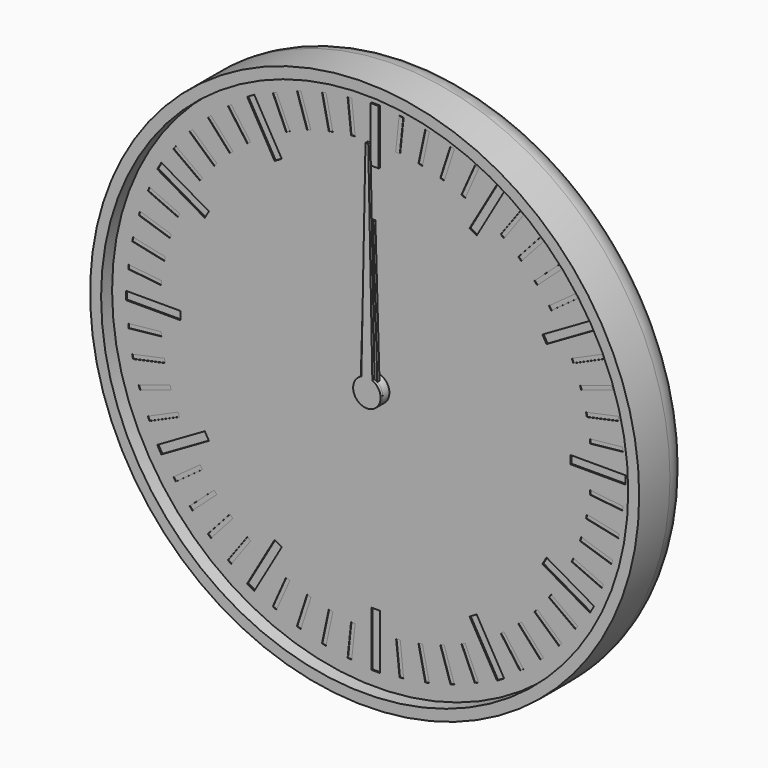
from build123d import *

# Parameters (mm, degrees)
F0_R      = 100
F1_DEPTH  = 24
F2_R      = 10
F3_T      = -4
F4_R      = 5
F4_R_2    = 3
F5_DEPTH  = 2
F6_DEPTH  = 19
F7_DEPTH  = 8
F9_DEPTH  = 4
F11_DEPTH = 4
F12_R     = 5
F12_R_2   = 3
F13_DEPTH = 2
F14_R     = 3
F15_DEPTH = 4
F17_DEPTH = 4
F18_R     = 3
F19_DEPTH = 2
F20_R     = 98
F20_R_2   = 5
F21_DEPTH = 1
F23_R     = 5
F23_R_2   = 3
F24_DEPTH = 2
F25_W     = 3
F25_H     = 20
F25_W_2   = 20
F25_H_2   = 3
F26_DEPTH = 0.5
F27_W     = 1.5
F27_H     = 12
F27_W_2   = 12
F27_H_2   = 1.5
F28_DEPTH = 0.2
F29_DEPTH = 1
F30_DEPTH = 0.4
F31_R     = 5
F31_R_2   = 3
F32_DEPTH = 5
F33_R     = 3
F34_DEPTH = 1
F36_DEPTH = 1


with BuildPart() as f1:
    # F0 (on Front) → F1 (new body)
    with BuildSketch(Plane.XZ):
        Circle(F0_R)
    extrude(amount=F1_DEPTH)

    # F2
    f2_edges = [f1.edges().sort_by_distance(p)[0] for p in [
        (-100, 0, 0),
    ]]
    fillet(f2_edges, radius=F2_R)

    # F3
    f3_openings = [f1.faces().sort_by_distance(p)[0] for p in [
        (0, -24, 0),
    ]]
    offset(amount=F3_T, openings=f3_openings)

    # F4 (on face) → F5 (join)
    with BuildSketch(Plane.XZ.offset(4)):
        Circle(F4_R)
        Circle(F4_R_2, mode=Mode.SUBTRACT)
        with Locations((40, 0)):
            Circle(F4_R)
        with Locations((40, 0)):
            Circle(F4_R_2, mode=Mode.SUBTRACT)
    extrude(amount=F5_DEPTH)


with BuildPart() as f6:
    # F6 (new): a face of the model
    f6_faces = [f1.part.faces().sort_by_distance(p)[0] for p in [
        (0, -4, 0),
    ]]
    extrude(f6_faces, amount=F6_DEPTH)

    # F8 (on face) → F9 (join)
    with BuildSketch(Plane.XZ.offset(6)):
        with BuildLine():
            ThreePointArc((9.2729637667, -1.3794085621), (9.3494561423, -0.6915886375), (9.375, 0))
            ThreePointArc((9.375, 0), (9.3494561423, 0.6915886375), (9.2729637667, 1.3794085621))
            ThreePointArc((9.2729637667, 1.3794085621), (8.9161548403, 2.8970343223), (8.3127812852, 4.3345463782))
            ThreePointArc((8.3127812852, 4.3345463782), (7.5845343223, 5.5104867402), (6.6911892658, 6.566476316))
            ThreePointArc((6.6911892658, 6.566476316), (5.5104867402, 7.5845343223), (4.1773988938, 8.3928519278))
            ThreePointArc((4.1773988938, 8.3928519278), (2.8970343223, 8.9161548403), (1.5536078905, 9.2453733036))
            ThreePointArc((1.5536078905, 9.2453733036), (0, 9.375), (-1.5536078905, 9.2453733036))
            ThreePointArc((-1.5536078905, 9.2453733036), (-2.8970343223, 8.9161548403), (-4.1773988938, 8.3928519278))
            ThreePointArc((-4.1773988938, 8.3928519278), (-5.5104867402, 7.5845343223), (-6.6911892658, 6.566476316))
            ThreePointArc((-6.6911892658, 6.566476316), (-7.5845343223, 5.5104867402), (-8.3127812852, 4.3345463782))
            ThreePointArc((-8.3127812852, 4.3345463782), (-8.9161548403, 2.8970343223), (-9.2729637667, 1.3794085621))
            ThreePointArc((-9.2729637667, 1.3794085621), (-9.375, 0), (-9.2729637667, -1.3794085621))
            ThreePointArc((-9.2729637667, -1.3794085621), (-8.9161548403, -2.8970343223), (-8.3127812852, -4.3345463782))
            ThreePointArc((-8.3127812852, -4.3345463782), (-7.5845343223, -5.5104867402), (-6.6911892658, -6.566476316))
            ThreePointArc((-6.6911892658, -6.566476316), (-5.5104867402, -7.5845343223), (-4.1773988938, -8.3928519278))
            ThreePointArc((-4.1773988938, -8.3928519278), (-2.8970343223, -8.9161548403), (-1.5536078905, -9.2453733036))
            ThreePointArc((-1.5536078905, -9.2453733036), (0, -9.375), (1.5536078905, -9.2453733036))
            ThreePointArc((1.5536078905, -9.2453733036), (2.8970343223, -8.9161548403), (4.1773988938, -8.3928519278))
            ThreePointArc((4.1773988938, -8.3928519278), (5.5104867402, -7.5845343223), (6.6911892658, -6.566476316))
            ThreePointArc((6.6911892658, -6.566476316), (7.5845343223, -5.5104867402), (8.3127812852, -4.3345463782))
            ThreePointArc((8.3127812852, -4.3345463782), (8.9161548403, -2.8970343223), (9.2729637667, -1.3794085621))
        make_face()
        with BuildLine():
            ThreePointArc((8.3127812852, 4.3345463782), (8.9161548403, 2.8970343223), (9.2729637667, 1.3794085621))
            Line((9.2729637667, 1.3794085621), (11.1823199426, 2.3946312492))
            Line((11.1823199426, 2.3946312492), (10.8182678729, 3.515068311))
            Line((10.8182678729, 3.515068311), (10.4542158031, 4.6355053728))
            Line((10.4542158031, 4.6355053728), (8.3127812852, 4.3345463782))
        make_face()
        with BuildLine():
            Line((11.1823199426, -2.3946312492), (9.2729637667, -1.3794085621))
            ThreePointArc((9.2729637667, -1.3794085621), (8.9161548403, -2.8970343223), (8.3127812852, -4.3345463782))
            Line((8.3127812852, -4.3345463782), (10.4542158031, -4.6355053728))
            Line((10.4542158031, -4.6355053728), (10.8182678729, -3.515068311))
            Line((10.8182678729, -3.515068311), (11.1823199426, -2.3946312492))
        make_face()
        with BuildLine():
            ThreePointArc((4.1773988938, 8.3928519278), (5.5104867402, 7.5845343223), (6.6911892658, 6.566476316))
            Line((6.6911892658, 6.566476316), (7.6391579371, 8.5101001246))
            Line((7.6391579371, 8.5101001246), (6.6860572448, 9.202568311))
            Line((6.6860572448, 9.202568311), (5.7329565525, 9.8950364974))
            Line((5.7329565525, 9.8950364974), (4.1773988938, 8.3928519278))
        make_face()
        with BuildLine():
            Line((7.6391579371, -8.5101001246), (6.6911892658, -6.566476316))
            ThreePointArc((6.6911892658, -6.566476316), (5.5104867402, -7.5845343223), (4.1773988938, -8.3928519278))
            Line((4.1773988938, -8.3928519278), (5.7329565525, -9.8950364974))
            Line((5.7329565525, -9.8950364974), (6.6860572448, -9.202568311))
            Line((6.6860572448, -9.202568311), (7.6391579371, -8.5101001246))
        make_face()
        with BuildLine():
            ThreePointArc((-1.5536078905, 9.2453733036), (0, 9.375), (1.5536078905, 9.2453733036))
            Line((1.5536078905, 9.2453733036), (1.1780972451, 11.375))
            Line((1.1780972451, 11.375), (0, 11.375))
            Line((0, 11.375), (-1.1780972451, 11.375))
            Line((-1.1780972451, 11.375), (-1.5536078905, 9.2453733036))
        make_face()
        with BuildLine():
            Line((1.1780972451, -11.375), (1.5536078905, -9.2453733036))
            ThreePointArc((1.5536078905, -9.2453733036), (0, -9.375), (-1.5536078905, -9.2453733036))
            Line((-1.5536078905, -9.2453733036), (-1.1780972451, -11.375))
            Line((-1.1780972451, -11.375), (0, -11.375))
            Line((0, -11.375), (1.1780972451, -11.375))
        make_face()
        with BuildLine():
            ThreePointArc((-6.6911892658, 6.566476316), (-5.5104867402, 7.5845343223), (-4.1773988938, 8.3928519278))
            Line((-4.1773988938, 8.3928519278), (-5.7329565525, 9.8950364974))
            Line((-5.7329565525, 9.8950364974), (-6.6860572448, 9.202568311))
            Line((-6.6860572448, 9.202568311), (-7.6391579371, 8.5101001246))
            Line((-7.6391579371, 8.5101001246), (-6.6911892658, 6.566476316))
        make_face()
        with BuildLine():
            Line((-5.7329565525, -9.8950364974), (-4.1773988938, -8.3928519278))
            ThreePointArc((-4.1773988938, -8.3928519278), (-5.5104867402, -7.5845343223), (-6.6911892658, -6.566476316))
            Line((-6.6911892658, -6.566476316), (-7.6391579371, -8.5101001246))
            Line((-7.6391579371, -8.5101001246), (-6.6860572448, -9.202568311))
            Line((-6.6860572448, -9.202568311), (-5.7329565525, -9.8950364974))
        make_face()
        with BuildLine():
            ThreePointArc((-9.2729637667, 1.3794085621), (-8.9161548403, 2.8970343223), (-8.3127812852, 4.3345463782))
            Line((-8.3127812852, 4.3345463782), (-10.4542158031, 4.6355053728))
            Line((-10.4542158031, 4.6355053728), (-10.8182678729, 3.515068311))
            Line((-10.8182678729, 3.515068311), (-11.1823199426, 2.3946312492))
            Line((-11.1823199426, 2.3946312492), (-9.2729637667, 1.3794085621))
        make_face()
        with BuildLine():
            Line((-10.4542158031, -4.6355053728), (-8.3127812852, -4.3345463782))
            ThreePointArc((-8.3127812852, -4.3345463782), (-8.9161548403, -2.8970343223), (-9.2729637667, -1.3794085621))
            Line((-9.2729637667, -1.3794085621), (-11.1823199426, -2.3946312492))
            Line((-11.1823199426, -2.3946312492), (-10.8182678729, -3.515068311))
            Line((-10.8182678729, -3.515068311), (-10.4542158031, -4.6355053728))
        make_face()
    extrude(amount=F9_DEPTH)

    # F35 (on face) → F36 (join)
    with BuildSketch(Plane.XZ.offset(23)):
        with BuildLine():
            ThreePointArc((-2, 4.582575695), (-2.7386127875, -4.1833001327), (5, 0))
            ThreePointArc((5, 0), (4.1833001327, 2.7386127875), (2, 4.582575695))
            ThreePointArc((2, 4.582575695), (0, 5), (-2, 4.582575695))
        make_face()
        with BuildLine():
            ThreePointArc((-2, 4.582575695), (0, 5), (2, 4.582575695))
            Line((2, 4.582575695), (0.5, 80))
            Line((0.5, 80), (0, 80))
            Line((0, 80), (-0.5, 80))
            Line((-0.5, 80), (-2, 4.582575695))
        make_face()
    extrude(amount=-F36_DEPTH)


with BuildPart() as f7:
    # F7 (new): a face of the model
    f7_faces = [f1.part.faces().sort_by_distance(p)[0] for p in [
        (40, -4, 0),
    ]]
    extrude(f7_faces, amount=F7_DEPTH)

    # F10 (on face) → F11 (join)
    with BuildSketch(Plane.XZ.offset(6)):
        with BuildLine():
            ThreePointArc((68.0829066802, -1.5381733945), (68.1144747006, -0.7693746225), (68.125, 0))
            ThreePointArc((68.125, 0), (68.1144747006, 0.7693746225), (68.0829066802, 1.5381733945))
            ThreePointArc((68.0829066802, 1.5381733945), (67.9709283072, 2.9398630294), (67.7890320221, 4.3342039956))
            ThreePointArc((67.7890320221, 4.3342039956), (67.5104012706, 5.8475163042), (67.1494235596, 7.3433252263))
            ThreePointArc((67.1494235596, 7.3433252263), (66.7484645208, 8.6911029668), (66.280643318, 10.0171558733))
            ThreePointArc((66.280643318, 10.0171558733), (65.6934659962, 11.4394680865), (65.0293803521, 12.8275385085))
            ThreePointArc((65.0293803521, 12.8275385085), (64.3569644814, 14.0625), (63.6236643925, 15.2623099717))
            ThreePointArc((63.6236643925, 15.2623099717), (62.7536029668, 16.5314602207), (61.815433119, 17.7511268046))
            ThreePointArc((61.815433119, 17.7511268046), (60.9009482166, 18.8192983038), (59.934217974, 19.8404278876))
            ThreePointArc((59.934217974, 19.8404278876), (58.8192983038, 20.9009482166), (57.6480467764, 21.8989056799))
            ThreePointArc((57.6480467764, 21.8989056799), (56.5314602207, 22.7536029668), (55.3735505752, 23.5514238999))
            ThreePointArc((55.3735505752, 23.5514238999), (54.0625, 24.3569644814), (52.709356105, 25.0895972944))
            ThreePointArc((52.709356105, 25.0895972944), (51.4394680865, 25.6934659962), (50.1409852457, 26.2331096755))
            ThreePointArc((50.1409852457, 26.2331096755), (48.6911029668, 26.7484645208), (47.2152055856, 27.1837531139))
            ThreePointArc((47.2152055856, 27.1837531139), (45.8475163042, 27.5104012706), (44.4652101991, 27.7682826779))
            ThreePointArc((44.4652101991, 27.7682826779), (42.9398630294, 27.9709283072), (41.4057159597, 28.0898484802))
            ThreePointArc((41.4057159597, 28.0898484802), (40, 28.125), (38.5942840403, 28.0898484802))
            ThreePointArc((38.5942840403, 28.0898484802), (37.0601369706, 27.9709283072), (35.5347898009, 27.7682826779))
            ThreePointArc((35.5347898009, 27.7682826779), (34.1524836958, 27.5104012706), (32.7847944144, 27.1837531139))
            ThreePointArc((32.7847944144, 27.1837531139), (31.3088970332, 26.7484645208), (29.8590147543, 26.2331096755))
            ThreePointArc((29.8590147543, 26.2331096755), (28.5605319135, 25.6934659962), (27.290643895, 25.0895972944))
            ThreePointArc((27.290643895, 25.0895972944), (25.9375, 24.3569644814), (24.6264494248, 23.5514238999))
            ThreePointArc((24.6264494248, 23.5514238999), (23.4685397793, 22.7536029668), (22.3519532236, 21.8989056799))
            ThreePointArc((22.3519532236, 21.8989056799), (21.1807016962, 20.9009482166), (20.065782026, 19.8404278876))
            ThreePointArc((20.065782026, 19.8404278876), (19.0990517834, 18.8192983038), (18.184566881, 17.7511268046))
            ThreePointArc((18.184566881, 17.7511268046), (17.2463970332, 16.5314602207), (16.3763356075, 15.2623099717))
            ThreePointArc((16.3763356075, 15.2623099717), (15.6430355186, 14.0625), (14.9706196479, 12.8275385085))
            ThreePointArc((14.9706196479, 12.8275385085), (14.3065340038, 11.4394680865), (13.719356682, 10.0171558733))
            ThreePointArc((13.719356682, 10.0171558733), (13.2515354792, 8.6911029668), (12.8505764404, 7.3433252263))
            ThreePointArc((12.8505764404, 7.3433252263), (12.4895987294, 5.8475163042), (12.2109679779, 4.3342039956))
            ThreePointArc((12.2109679779, 4.3342039956), (12.0290716928, 2.9398630294), (11.9170933198, 1.5381733945))
            ThreePointArc((11.9170933198, 1.5381733945), (11.875, 0), (11.9170933198, -1.5381733945))
            ThreePointArc((11.9170933198, -1.5381733945), (12.0290716928, -2.9398630294), (12.2109679779, -4.3342039956))
            ThreePointArc((12.2109679779, -4.3342039956), (12.4895987294, -5.8475163042), (12.8505764404, -7.3433252263))
            ThreePointArc((12.8505764404, -7.3433252263), (13.2515354792, -8.6911029668), (13.719356682, -10.0171558733))
            ThreePointArc((13.719356682, -10.0171558733), (14.3065340038, -11.4394680865), (14.9706196479, -12.8275385085))
            ThreePointArc((14.9706196479, -12.8275385085), (15.6430355186, -14.0625), (16.3763356075, -15.2623099717))
            ThreePointArc((16.3763356075, -15.2623099717), (17.2463970332, -16.5314602207), (18.184566881, -17.7511268046))
            ThreePointArc((18.184566881, -17.7511268046), (19.0990517834, -18.8192983038), (20.065782026, -19.8404278876))
            ThreePointArc((20.065782026, -19.8404278876), (21.1807016962, -20.9009482166), (22.3519532236, -21.8989056799))
            ThreePointArc((22.3519532236, -21.8989056799), (23.4685397793, -22.7536029668), (24.6264494248, -23.5514238999))
            ThreePointArc((24.6264494248, -23.5514238999), (25.9375, -24.3569644814), (27.290643895, -25.0895972944))
            ThreePointArc((27.290643895, -25.0895972944), (28.5605319135, -25.6934659962), (29.8590147543, -26.2331096755))
            ThreePointArc((29.8590147543, -26.2331096755), (31.3088970332, -26.7484645208), (32.7847944144, -27.1837531139))
            ThreePointArc((32.7847944144, -27.1837531139), (34.1524836958, -27.5104012706), (35.5347898009, -27.7682826779))
            ThreePointArc((35.5347898009, -27.7682826779), (37.0601369706, -27.9709283072), (38.5942840403, -28.0898484802))
            ThreePointArc((38.5942840403, -28.0898484802), (40, -28.125), (41.4057159597, -28.0898484802))
            ThreePointArc((41.4057159597, -28.0898484802), (42.9398630294, -27.9709283072), (44.4652101991, -27.7682826779))
            ThreePointArc((44.4652101991, -27.7682826779), (45.8475163042, -27.5104012706), (47.2152055856, -27.1837531139))
            ThreePointArc((47.2152055856, -27.1837531139), (48.6911029668, -26.7484645208), (50.1409852457, -26.2331096755))
            ThreePointArc((50.1409852457, -26.2331096755), (51.4394680865, -25.6934659962), (52.709356105, -25.0895972944))
            ThreePointArc((52.709356105, -25.0895972944), (54.0625, -24.3569644814), (55.3735505752, -23.5514238999))
            ThreePointArc((55.3735505752, -23.5514238999), (56.5314602207, -22.7536029668), (57.6480467764, -21.8989056799))
            ThreePointArc((57.6480467764, -21.8989056799), (58.8192983038, -20.9009482166), (59.934217974, -19.8404278876))
            ThreePointArc((59.934217974, -19.8404278876), (60.9009482166, -18.8192983038), (61.815433119, -17.7511268046))
            ThreePointArc((61.815433119, -17.7511268046), (62.7536029668, -16.5314602207), (63.6236643925, -15.2623099717))
            ThreePointArc((63.6236643925, -15.2623099717), (64.3569644814, -14.0625), (65.0293803521, -12.8275385085))
            ThreePointArc((65.0293803521, -12.8275385085), (65.6934659962, -11.4394680865), (66.280643318, -10.0171558733))
            ThreePointArc((66.280643318, -10.0171558733), (66.7484645208, -8.6911029668), (67.1494235596, -7.3433252263))
            ThreePointArc((67.1494235596, -7.3433252263), (67.5104012706, -5.8475163042), (67.7890320221, -4.3342039956))
            ThreePointArc((67.7890320221, -4.3342039956), (67.9709283072, -2.9398630294), (68.0829066802, -1.5381733945))
        make_face()
        with BuildLine():
            ThreePointArc((68.0829066802, 1.5381733945), (68.1144747006, 0.7693746225), (68.125, 0))
            ThreePointArc((68.125, 0), (68.1144747006, -0.7693746225), (68.0829066802, -1.5381733945))
            Line((68.0829066802, -1.5381733945), (70.125, -1.1780972451))
            Line((70.125, -1.1780972451), (70.125, 0))
            Line((70.125, 0), (70.125, 1.1780972451))
            Line((70.125, 1.1780972451), (68.0829066802, 1.5381733945))
        make_face()
        with BuildLine():
            ThreePointArc((67.1494235596, 7.3433252263), (67.5104012706, 5.8475163042), (67.7890320221, 4.3342039956))
            Line((67.7890320221, 4.3342039956), (69.7116366623, 5.1109866922))
            Line((69.7116366623, 5.1109866922), (69.4666964721, 6.2633396859))
            Line((69.4666964721, 6.2633396859), (69.2217562819, 7.4156926796))
            Line((69.2217562819, 7.4156926796), (67.1494235596, 7.3433252263))
        make_face()
        with BuildLine():
            Line((69.7116366623, -5.1109866922), (67.7890320221, -4.3342039956))
            ThreePointArc((67.7890320221, -4.3342039956), (67.5104012706, -5.8475163042), (67.1494235596, -7.3433252263))
            Line((67.1494235596, -7.3433252263), (69.2217562819, -7.4156926796))
            Line((69.2217562819, -7.4156926796), (69.4666964721, -6.2633396859))
            Line((69.4666964721, -6.2633396859), (69.7116366623, -5.1109866922))
        make_face()
        with BuildLine():
            ThreePointArc((65.0293803521, 12.8275385085), (65.6934659962, 11.4394680865), (66.280643318, 10.0171558733))
            Line((66.280643318, 10.0171558733), (67.9997322302, 11.1766959857))
            Line((67.9997322302, 11.1766959857), (67.5205569115, 12.2529413727))
            Line((67.5205569115, 12.2529413727), (67.0413815928, 13.3291867596))
            Line((67.0413815928, 13.3291867596), (65.0293803521, 12.8275385085))
        make_face()
        with BuildLine():
            Line((67.9997322302, -11.1766959857), (66.280643318, -10.0171558733))
            ThreePointArc((66.280643318, -10.0171558733), (65.6934659962, -11.4394680865), (65.0293803521, -12.8275385085))
            Line((65.0293803521, -12.8275385085), (67.0413815928, -13.3291867596))
            Line((67.0413815928, -13.3291867596), (67.5205569115, -12.2529413727))
            Line((67.5205569115, -12.2529413727), (67.9997322302, -11.1766959857))
        make_face()
        with BuildLine():
            ThreePointArc((61.815433119, 17.7511268046), (62.7536029668, 16.5314602207), (63.6236643925, 15.2623099717))
            Line((63.6236643925, 15.2623099717), (65.064105142, 16.753930033))
            Line((65.064105142, 16.753930033), (64.3716369555, 17.7070307253))
            Line((64.3716369555, 17.7070307253), (63.6791687691, 18.6601314176))
            Line((63.6791687691, 18.6601314176), (61.815433119, 17.7511268046))
        make_face()
        with BuildLine():
            Line((65.064105142, -16.753930033), (63.6236643925, -15.2623099717))
            ThreePointArc((63.6236643925, -15.2623099717), (62.7536029668, -16.5314602207), (61.815433119, -17.7511268046))
            Line((61.815433119, -17.7511268046), (63.6791687691, -18.6601314176))
            Line((63.6791687691, -18.6601314176), (64.3716369555, -17.7070307253))
            Line((64.3716369555, -17.7070307253), (65.064105142, -16.753930033))
        make_face()
        with BuildLine():
            ThreePointArc((57.6480467764, 21.8989056799), (58.8192983038, 20.9009482166), (59.934217974, 19.8404278876))
            Line((59.934217974, 19.8404278876), (61.0330563882, 21.5989369435))
            Line((61.0330563882, 21.5989369435), (60.1575595166, 22.3872378675))
            Line((60.1575595166, 22.3872378675), (59.282062645, 23.1755387915))
            Line((59.282062645, 23.1755387915), (57.6480467764, 21.8989056799))
        make_face()
        with BuildLine():
            Line((61.0330563882, -21.5989369435), (59.934217974, -19.8404278876))
            ThreePointArc((59.934217974, -19.8404278876), (58.8192983038, -20.9009482166), (57.6480467764, -21.8989056799))
            Line((57.6480467764, -21.8989056799), (59.282062645, -23.1755387915))
            Line((59.282062645, -23.1755387915), (60.1575595166, -22.3872378675))
            Line((60.1575595166, -22.3872378675), (61.0330563882, -21.5989369435))
        make_face()
        with BuildLine():
            ThreePointArc((52.709356105, 25.0895972944), (54.0625, 24.3569644814), (55.3735505752, 23.5514238999))
            Line((55.3735505752, 23.5514238999), (56.0827621424, 25.4999666665))
            Line((56.0827621424, 25.4999666665), (55.0625, 26.089015289))
            Line((55.0625, 26.089015289), (54.0422378576, 26.6780639116))
            Line((54.0422378576, 26.6780639116), (52.709356105, 25.0895972944))
        make_face()
        with BuildLine():
            Line((56.0827621424, -25.4999666665), (55.3735505752, -23.5514238999))
            ThreePointArc((55.3735505752, -23.5514238999), (54.0625, -24.3569644814), (52.709356105, -25.0895972944))
            Line((52.709356105, -25.0895972944), (54.0422378576, -26.6780639116))
            Line((54.0422378576, -26.6780639116), (55.0625, -26.089015289))
            Line((55.0625, -26.089015289), (56.0827621424, -25.4999666665))
        make_face()
        with BuildLine():
            ThreePointArc((47.2152055856, 27.1837531139), (48.6911029668, 26.7484645208), (50.1409852457, 26.2331096755))
            Line((50.1409852457, 26.2331096755), (50.4295740173, 28.2865254836))
            Line((50.4295740173, 28.2865254836), (49.3091369555, 28.6505775534))
            Line((49.3091369555, 28.6505775534), (48.1886998938, 29.0146296232))
            Line((48.1886998938, 29.0146296232), (47.2152055856, 27.1837531139))
        make_face()
        with BuildLine():
            Line((50.4295740173, -28.2865254836), (50.1409852457, -26.2331096755))
            ThreePointArc((50.1409852457, -26.2331096755), (48.6911029668, -26.7484645208), (47.2152055856, -27.1837531139))
            Line((47.2152055856, -27.1837531139), (48.1886998938, -29.0146296232))
            Line((48.1886998938, -29.0146296232), (49.3091369555, -28.6505775534))
            Line((49.3091369555, -28.6505775534), (50.4295740173, -28.2865254836))
        make_face()
        with BuildLine():
            ThreePointArc((41.4057159597, 28.0898484802), (42.9398630294, 27.9709283072), (44.4652101991, 27.7682826779))
            Line((44.4652101991, 27.7682826779), (44.3205634611, 29.8368274034))
            Line((44.3205634611, 29.8368274034), (43.1489199559, 29.959972098))
            Line((43.1489199559, 29.959972098), (41.9772764508, 30.0831167926))
            Line((41.9772764508, 30.0831167926), (41.4057159597, 28.0898484802))
        make_face()
        with BuildLine():
            Line((44.3205634611, -29.8368274034), (44.4652101991, -27.7682826779))
            ThreePointArc((44.4652101991, -27.7682826779), (42.9398630294, -27.9709283072), (41.4057159597, -28.0898484802))
            Line((41.4057159597, -28.0898484802), (41.9772764508, -30.0831167926))
            Line((41.9772764508, -30.0831167926), (43.1489199559, -29.959972098))
            Line((43.1489199559, -29.959972098), (44.3205634611, -29.8368274034))
        make_face()
        with BuildLine():
            ThreePointArc((35.5347898009, 27.7682826779), (37.0601369706, 27.9709283072), (38.5942840403, 28.0898484802))
            Line((38.5942840403, 28.0898484802), (38.0227235492, 30.0831167926))
            Line((38.0227235492, 30.0831167926), (36.8510800441, 29.959972098))
            Line((36.8510800441, 29.959972098), (35.6794365389, 29.8368274034))
            Line((35.6794365389, 29.8368274034), (35.5347898009, 27.7682826779))
        make_face()
        with BuildLine():
            Line((38.0227235492, -30.0831167926), (38.5942840403, -28.0898484802))
            ThreePointArc((38.5942840403, -28.0898484802), (37.0601369706, -27.9709283072), (35.5347898009, -27.7682826779))
            Line((35.5347898009, -27.7682826779), (35.6794365389, -29.8368274034))
            Line((35.6794365389, -29.8368274034), (36.8510800441, -29.959972098))
            Line((36.8510800441, -29.959972098), (38.0227235492, -30.0831167926))
        make_face()
        with BuildLine():
            ThreePointArc((29.8590147543, 26.2331096755), (31.3088970332, 26.7484645208), (32.7847944144, 27.1837531139))
            Line((32.7847944144, 27.1837531139), (31.8113001062, 29.0146296232))
            Line((31.8113001062, 29.0146296232), (30.6908630445, 28.6505775534))
            Line((30.6908630445, 28.6505775534), (29.5704259827, 28.2865254836))
            Line((29.5704259827, 28.2865254836), (29.8590147543, 26.2331096755))
        make_face()
        with BuildLine():
            Line((31.8113001062, -29.0146296232), (32.7847944144, -27.1837531139))
            ThreePointArc((32.7847944144, -27.1837531139), (31.3088970332, -26.7484645208), (29.8590147543, -26.2331096755))
            Line((29.8590147543, -26.2331096755), (29.5704259827, -28.2865254836))
            Line((29.5704259827, -28.2865254836), (30.6908630445, -28.6505775534))
            Line((30.6908630445, -28.6505775534), (31.8113001062, -29.0146296232))
        make_face()
        with BuildLine():
            ThreePointArc((24.6264494248, 23.5514238999), (25.9375, 24.3569644814), (27.290643895, 25.0895972944))
            Line((27.290643895, 25.0895972944), (25.9577621424, 26.6780639116))
            Line((25.9577621424, 26.6780639116), (24.9375, 26.089015289))
            Line((24.9375, 26.089015289), (23.9172378576, 25.4999666665))
            Line((23.9172378576, 25.4999666665), (24.6264494248, 23.5514238999))
        make_face()
        with BuildLine():
            Line((25.9577621424, -26.6780639116), (27.290643895, -25.0895972944))
            ThreePointArc((27.290643895, -25.0895972944), (25.9375, -24.3569644814), (24.6264494248, -23.5514238999))
            Line((24.6264494248, -23.5514238999), (23.9172378576, -25.4999666665))
            Line((23.9172378576, -25.4999666665), (24.9375, -26.089015289))
            Line((24.9375, -26.089015289), (25.9577621424, -26.6780639116))
        make_face()
        with BuildLine():
            ThreePointArc((20.065782026, 19.8404278876), (21.1807016962, 20.9009482166), (22.3519532236, 21.8989056799))
            Line((22.3519532236, 21.8989056799), (20.717937355, 23.1755387915))
            Line((20.717937355, 23.1755387915), (19.8424404834, 22.3872378675))
            Line((19.8424404834, 22.3872378675), (18.9669436118, 21.5989369435))
            Line((18.9669436118, 21.5989369435), (20.065782026, 19.8404278876))
        make_face()
        with BuildLine():
            Line((20.717937355, -23.1755387915), (22.3519532236, -21.8989056799))
            ThreePointArc((22.3519532236, -21.8989056799), (21.1807016962, -20.9009482166), (20.065782026, -19.8404278876))
            Line((20.065782026, -19.8404278876), (18.9669436118, -21.5989369435))
            Line((18.9669436118, -21.5989369435), (19.8424404834, -22.3872378675))
            Line((19.8424404834, -22.3872378675), (20.717937355, -23.1755387915))
        make_face()
        with BuildLine():
            ThreePointArc((16.3763356075, 15.2623099717), (17.2463970332, 16.5314602207), (18.184566881, 17.7511268046))
            Line((18.184566881, 17.7511268046), (16.3208312309, 18.6601314176))
            Line((16.3208312309, 18.6601314176), (15.6283630445, 17.7070307253))
            Line((15.6283630445, 17.7070307253), (14.935894858, 16.753930033))
            Line((14.935894858, 16.753930033), (16.3763356075, 15.2623099717))
        make_face()
        with BuildLine():
            Line((16.3208312309, -18.6601314176), (18.184566881, -17.7511268046))
            ThreePointArc((18.184566881, -17.7511268046), (17.2463970332, -16.5314602207), (16.3763356075, -15.2623099717))
            Line((16.3763356075, -15.2623099717), (14.935894858, -16.753930033))
            Line((14.935894858, -16.753930033), (15.6283630445, -17.7070307253))
            Line((15.6283630445, -17.7070307253), (16.3208312309, -18.6601314176))
        make_face()
        with BuildLine():
            ThreePointArc((13.719356682, 10.0171558733), (14.3065340038, 11.4394680865), (14.9706196479, 12.8275385085))
            Line((14.9706196479, 12.8275385085), (12.9586184072, 13.3291867596))
            Line((12.9586184072, 13.3291867596), (12.4794430885, 12.2529413727))
            Line((12.4794430885, 12.2529413727), (12.0002677698, 11.1766959857))
            Line((12.0002677698, 11.1766959857), (13.719356682, 10.0171558733))
        make_face()
        with BuildLine():
            Line((12.9586184072, -13.3291867596), (14.9706196479, -12.8275385085))
            ThreePointArc((14.9706196479, -12.8275385085), (14.3065340038, -11.4394680865), (13.719356682, -10.0171558733))
            Line((13.719356682, -10.0171558733), (12.0002677698, -11.1766959857))
            Line((12.0002677698, -11.1766959857), (12.4794430885, -12.2529413727))
            Line((12.4794430885, -12.2529413727), (12.9586184072, -13.3291867596))
        make_face()
        with BuildLine():
            ThreePointArc((12.2109679779, 4.3342039956), (12.4895987294, 5.8475163042), (12.8505764404, 7.3433252263))
            Line((12.8505764404, 7.3433252263), (10.7782437181, 7.4156926796))
            Line((10.7782437181, 7.4156926796), (10.5333035279, 6.2633396859))
            Line((10.5333035279, 6.2633396859), (10.2883633377, 5.1109866922))
            Line((10.2883633377, 5.1109866922), (12.2109679779, 4.3342039956))
        make_face()
        with BuildLine():
            Line((10.7782437181, -7.4156926796), (12.8505764404, -7.3433252263))
            ThreePointArc((12.8505764404, -7.3433252263), (12.4895987294, -5.8475163042), (12.2109679779, -4.3342039956))
            Line((12.2109679779, -4.3342039956), (10.2883633377, -5.1109866922))
            Line((10.2883633377, -5.1109866922), (10.5333035279, -6.2633396859))
            Line((10.5333035279, -6.2633396859), (10.7782437181, -7.4156926796))
        make_face()
        with BuildLine():
            ThreePointArc((11.9170933198, -1.5381733945), (11.875, 0), (11.9170933198, 1.5381733945))
            Line((11.9170933198, 1.5381733945), (9.875, 1.1780972451))
            Line((9.875, 1.1780972451), (9.875, 0))
            Line((9.875, 0), (9.875, -1.1780972451))
            Line((9.875, -1.1780972451), (11.9170933198, -1.5381733945))
        make_face()
    extrude(amount=F11_DEPTH)

    # F16 (on face) → F17 (join)
    with BuildSketch(Plane.XZ.offset(12)):
        with BuildLine():
            ThreePointArc((47.4288750323, -1.0304444454), (47.4821976298, -0.5164480894), (47.5, 0))
            ThreePointArc((47.5, 0), (47.4821976298, 0.5164480894), (47.4288750323, 1.0304444454))
            ThreePointArc((47.4288750323, 1.0304444454), (47.1329238722, 2.3176274578), (46.6157661985, 3.532936117))
            ThreePointArc((46.6157661985, 3.532936117), (46.0676274578, 4.4083893922), (45.4044061018, 5.2002302532))
            ThreePointArc((45.4044061018, 5.2002302532), (44.4083893922, 6.0676274578), (43.2756595386, 6.7468551628))
            ThreePointArc((43.2756595386, 6.7468551628), (42.3176274578, 7.1329238722), (41.3156377295, 7.3837048536))
            ThreePointArc((41.3156377295, 7.3837048536), (40, 7.5), (38.6843622705, 7.3837048536))
            ThreePointArc((38.6843622705, 7.3837048536), (37.6823725422, 7.1329238722), (36.7243404614, 6.7468551628))
            ThreePointArc((36.7243404614, 6.7468551628), (35.5916106078, 6.0676274578), (34.5955938982, 5.2002302532))
            ThreePointArc((34.5955938982, 5.2002302532), (33.9323725422, 4.4083893922), (33.3842338015, 3.532936117))
            ThreePointArc((33.3842338015, 3.532936117), (32.8670761278, 2.3176274578), (32.5711249677, 1.0304444454))
            ThreePointArc((32.5711249677, 1.0304444454), (32.5, 0), (32.5711249677, -1.0304444454))
            ThreePointArc((32.5711249677, -1.0304444454), (32.8670761278, -2.3176274578), (33.3842338015, -3.532936117))
            ThreePointArc((33.3842338015, -3.532936117), (33.9323725422, -4.4083893922), (34.5955938982, -5.2002302532))
            ThreePointArc((34.5955938982, -5.2002302532), (35.5916106078, -6.0676274578), (36.7243404614, -6.7468551628))
            ThreePointArc((36.7243404614, -6.7468551628), (37.6823725422, -7.1329238722), (38.6843622705, -7.3837048536))
            ThreePointArc((38.6843622705, -7.3837048536), (40, -7.5), (41.3156377295, -7.3837048536))
            ThreePointArc((41.3156377295, -7.3837048536), (42.3176274578, -7.1329238722), (43.2756595386, -6.7468551628))
            ThreePointArc((43.2756595386, -6.7468551628), (44.4083893922, -6.0676274578), (45.4044061018, -5.2002302532))
            ThreePointArc((45.4044061018, -5.2002302532), (46.0676274578, -4.4083893922), (46.6157661985, -3.532936117))
            ThreePointArc((46.6157661985, -3.532936117), (47.1329238722, -2.3176274578), (47.4288750323, -1.0304444454))
        make_face()
        with BuildLine():
            ThreePointArc((46.6157661985, 3.532936117), (47.1329238722, 2.3176274578), (47.4288750323, 1.0304444454))
            Line((47.4288750323, 1.0304444454), (49.3262785606, 2.0393117971))
            Line((49.3262785606, 2.0393117971), (48.743795249, 3.832011096))
            Line((48.743795249, 3.832011096), (46.6157661985, 3.532936117))
        make_face()
        with BuildLine():
            Line((49.3262785606, -2.0393117971), (47.4288750323, -1.0304444454))
            ThreePointArc((47.4288750323, -1.0304444454), (47.1329238722, -2.3176274578), (46.6157661985, -3.532936117))
            Line((46.6157661985, -3.532936117), (48.743795249, -3.832011096))
            Line((48.743795249, -3.832011096), (49.3262785606, -2.0393117971))
        make_face()
        with BuildLine():
            ThreePointArc((43.2756595386, 6.7468551628), (44.4083893922, 6.0676274578), (45.4044061018, 5.2002302532))
            Line((45.4044061018, 5.2002302532), (46.3464404506, 7.1316868974))
            Line((46.3464404506, 7.1316868974), (44.8214793429, 8.2396359957))
            Line((44.8214793429, 8.2396359957), (43.2756595386, 6.7468551628))
        make_face()
        with BuildLine():
            Line((46.3464404506, -7.1316868974), (45.4044061018, -5.2002302532))
            ThreePointArc((45.4044061018, -5.2002302532), (44.4083893922, -6.0676274578), (43.2756595386, -6.7468551628))
            Line((43.2756595386, -6.7468551628), (44.8214793429, -8.2396359957))
            Line((44.8214793429, -8.2396359957), (46.3464404506, -7.1316868974))
        make_face()
        with BuildLine():
            ThreePointArc((38.6843622705, 7.3837048536), (40, 7.5), (41.3156377295, 7.3837048536))
            Line((41.3156377295, 7.3837048536), (40.9424777961, 9.5))
            Line((40.9424777961, 9.5), (39.0575222039, 9.5))
            Line((39.0575222039, 9.5), (38.6843622705, 7.3837048536))
        make_face()
        with BuildLine():
            Line((40.9424777961, -9.5), (41.3156377295, -7.3837048536))
            ThreePointArc((41.3156377295, -7.3837048536), (40, -7.5), (38.6843622705, -7.3837048536))
            Line((38.6843622705, -7.3837048536), (39.0575222039, -9.5))
            Line((39.0575222039, -9.5), (40.9424777961, -9.5))
        make_face()
        with BuildLine():
            ThreePointArc((34.5955938982, 5.2002302532), (35.5916106078, 6.0676274578), (36.7243404614, 6.7468551628))
            Line((36.7243404614, 6.7468551628), (35.1785206571, 8.2396359957))
            Line((35.1785206571, 8.2396359957), (33.6535595494, 7.1316868974))
            Line((33.6535595494, 7.1316868974), (34.5955938982, 5.2002302532))
        make_face()
        with BuildLine():
            Line((35.1785206571, -8.2396359957), (36.7243404614, -6.7468551628))
            ThreePointArc((36.7243404614, -6.7468551628), (35.5916106078, -6.0676274578), (34.5955938982, -5.2002302532))
            Line((34.5955938982, -5.2002302532), (33.6535595494, -7.1316868974))
            Line((33.6535595494, -7.1316868974), (35.1785206571, -8.2396359957))
        make_face()
        with BuildLine():
            ThreePointArc((32.5711249677, 1.0304444454), (32.8670761278, 2.3176274578), (33.3842338015, 3.532936117))
            Line((33.3842338015, 3.532936117), (31.256204751, 3.832011096))
            Line((31.256204751, 3.832011096), (30.6737214394, 2.0393117971))
            Line((30.6737214394, 2.0393117971), (32.5711249677, 1.0304444454))
        make_face()
        with BuildLine():
            Line((31.256204751, -3.832011096), (33.3842338015, -3.532936117))
            ThreePointArc((33.3842338015, -3.532936117), (32.8670761278, -2.3176274578), (32.5711249677, -1.0304444454))
            Line((32.5711249677, -1.0304444454), (30.6737214394, -2.0393117971))
            Line((30.6737214394, -2.0393117971), (31.256204751, -3.832011096))
        make_face()
    extrude(amount=F17_DEPTH)

    # F18 (on face) → F19 (join)
    with BuildSketch(Plane.XZ.offset(16)):
        with Locations((40, 0)):
            Circle(F18_R)
    extrude(amount=F19_DEPTH)


with BuildPart() as f13:
    # F12 (on face) → F13 (new body)
    with BuildSketch(Plane.XZ.offset(10)):
        Circle(F12_R)
        Circle(F12_R_2, mode=Mode.SUBTRACT)
    extrude(amount=F13_DEPTH)

    # F14 (on face) → F15 (join)
    with BuildSketch(Plane.XZ.offset(12)):
        with BuildLine():
            ThreePointArc((29.9718156995, -1.3001014101), (29.9929530972, -0.6502034357), (30, 0))
            ThreePointArc((30, 0), (29.9929530972, 0.6502034357), (29.9718156995, 1.3001014101))
            ThreePointArc((29.9718156995, 1.3001014101), (29.907520012, 2.3537728718), (29.8061935814, 3.4045299509))
            ThreePointArc((29.8061935814, 3.4045299509), (29.6306502179, 4.6930339512), (29.3994322443, 5.9727199596))
            ThreePointArc((29.3994322443, 5.9727199596), (29.1710976119, 7.0033609157), (28.9066440563, 8.0253304855))
            ThreePointArc((28.9066440563, 8.0253304855), (28.5316954889, 9.2705098312), (28.1031371961, 10.4982703213))
            ThreePointArc((28.1031371961, 10.4982703213), (27.7163859753, 11.480502971), (27.2953170189, 12.448520749))
            ThreePointArc((27.2953170189, 12.448520749), (26.7301957257, 13.6197149922), (26.1148496411, 14.765318426))
            ThreePointArc((26.1148496411, 14.765318426), (25.5792049306, 15.6749569415), (25.0118886885, 16.5651871174))
            ThreePointArc((25.0118886885, 16.5651871174), (24.2705098312, 17.6335575688), (23.4835278178, 18.6687953878))
            ThreePointArc((23.4835278178, 18.6687953878), (22.812178968, 19.4834414499), (22.1125846489, 20.2739636023))
            ThreePointArc((22.1125846489, 20.2739636023), (21.2132034356, 21.2132034356), (20.2739636023, 22.1125846489))
            ThreePointArc((20.2739636023, 22.1125846489), (19.4834414499, 22.812178968), (18.6687953878, 23.4835278178))
            ThreePointArc((18.6687953878, 23.4835278178), (17.6335575688, 24.2705098312), (16.5651871174, 25.0118886885))
            ThreePointArc((16.5651871174, 25.0118886885), (15.6749569415, 25.5792049306), (14.765318426, 26.1148496411))
            ThreePointArc((14.765318426, 26.1148496411), (13.6197149922, 26.7301957257), (12.448520749, 27.2953170189))
            ThreePointArc((12.448520749, 27.2953170189), (11.480502971, 27.7163859753), (10.4982703213, 28.1031371961))
            ThreePointArc((10.4982703213, 28.1031371961), (9.2705098312, 28.5316954889), (8.0253304855, 28.9066440563))
            ThreePointArc((8.0253304855, 28.9066440563), (7.0033609157, 29.1710976119), (5.9727199596, 29.3994322443))
            ThreePointArc((5.9727199596, 29.3994322443), (4.6930339512, 29.6306502179), (3.4045299509, 29.8061935814))
            ThreePointArc((3.4045299509, 29.8061935814), (2.3537728718, 29.907520012), (1.3001014101, 29.9718156995))
            ThreePointArc((1.3001014101, 29.9718156995), (0, 30), (-1.3001014101, 29.9718156995))
            ThreePointArc((-1.3001014101, 29.9718156995), (-2.3537728718, 29.907520012), (-3.4045299509, 29.8061935814))
            ThreePointArc((-3.4045299509, 29.8061935814), (-4.6930339512, 29.6306502179), (-5.9727199596, 29.3994322443))
            ThreePointArc((-5.9727199596, 29.3994322443), (-7.0033609157, 29.1710976119), (-8.0253304855, 28.9066440563))
            ThreePointArc((-8.0253304855, 28.9066440563), (-9.2705098312, 28.5316954889), (-10.4982703213, 28.1031371961))
            ThreePointArc((-10.4982703213, 28.1031371961), (-11.480502971, 27.7163859753), (-12.448520749, 27.2953170189))
            ThreePointArc((-12.448520749, 27.2953170189), (-13.6197149922, 26.7301957257), (-14.765318426, 26.1148496411))
            ThreePointArc((-14.765318426, 26.1148496411), (-15.6749569415, 25.5792049306), (-16.5651871174, 25.0118886885))
            ThreePointArc((-16.5651871174, 25.0118886885), (-17.6335575688, 24.2705098312), (-18.6687953878, 23.4835278178))
            ThreePointArc((-18.6687953878, 23.4835278178), (-19.4834414499, 22.812178968), (-20.2739636023, 22.1125846489))
            ThreePointArc((-20.2739636023, 22.1125846489), (-21.2132034356, 21.2132034356), (-22.1125846489, 20.2739636023))
            ThreePointArc((-22.1125846489, 20.2739636023), (-22.812178968, 19.4834414499), (-23.4835278178, 18.6687953878))
            ThreePointArc((-23.4835278178, 18.6687953878), (-24.2705098312, 17.6335575688), (-25.0118886885, 16.5651871174))
            ThreePointArc((-25.0118886885, 16.5651871174), (-25.5792049306, 15.6749569415), (-26.1148496411, 14.765318426))
            ThreePointArc((-26.1148496411, 14.765318426), (-26.7301957257, 13.6197149922), (-27.2953170189, 12.448520749))
            ThreePointArc((-27.2953170189, 12.448520749), (-27.7163859753, 11.480502971), (-28.1031371961, 10.4982703213))
            ThreePointArc((-28.1031371961, 10.4982703213), (-28.5316954889, 9.2705098312), (-28.9066440563, 8.0253304855))
            ThreePointArc((-28.9066440563, 8.0253304855), (-29.1710976119, 7.0033609157), (-29.3994322443, 5.9727199596))
            ThreePointArc((-29.3994322443, 5.9727199596), (-29.6306502179, 4.6930339512), (-29.8061935814, 3.4045299509))
            ThreePointArc((-29.8061935814, 3.4045299509), (-29.907520012, 2.3537728718), (-29.9718156995, 1.3001014101))
            ThreePointArc((-29.9718156995, 1.3001014101), (-30, 0), (-29.9718156995, -1.3001014101))
            ThreePointArc((-29.9718156995, -1.3001014101), (-29.907520012, -2.3537728718), (-29.8061935814, -3.4045299509))
            ThreePointArc((-29.8061935814, -3.4045299509), (-29.6306502179, -4.6930339512), (-29.3994322443, -5.9727199596))
            ThreePointArc((-29.3994322443, -5.9727199596), (-29.1710976119, -7.0033609157), (-28.9066440563, -8.0253304855))
            ThreePointArc((-28.9066440563, -8.0253304855), (-28.5316954889, -9.2705098312), (-28.1031371961, -10.4982703213))
            ThreePointArc((-28.1031371961, -10.4982703213), (-27.7163859753, -11.480502971), (-27.2953170189, -12.448520749))
            ThreePointArc((-27.2953170189, -12.448520749), (-26.7301957257, -13.6197149922), (-26.1148496411, -14.765318426))
            ThreePointArc((-26.1148496411, -14.765318426), (-25.5792049306, -15.6749569415), (-25.0118886885, -16.5651871174))
            ThreePointArc((-25.0118886885, -16.5651871174), (-24.2705098312, -17.6335575688), (-23.4835278178, -18.6687953878))
            ThreePointArc((-23.4835278178, -18.6687953878), (-22.812178968, -19.4834414499), (-22.1125846489, -20.2739636023))
            ThreePointArc((-22.1125846489, -20.2739636023), (-21.2132034356, -21.2132034356), (-20.2739636023, -22.1125846489))
            ThreePointArc((-20.2739636023, -22.1125846489), (-19.4834414499, -22.812178968), (-18.6687953878, -23.4835278178))
            ThreePointArc((-18.6687953878, -23.4835278178), (-17.6335575688, -24.2705098312), (-16.5651871174, -25.0118886885))
            ThreePointArc((-16.5651871174, -25.0118886885), (-15.6749569415, -25.5792049306), (-14.765318426, -26.1148496411))
            ThreePointArc((-14.765318426, -26.1148496411), (-13.6197149922, -26.7301957257), (-12.448520749, -27.2953170189))
            ThreePointArc((-12.448520749, -27.2953170189), (-11.480502971, -27.7163859753), (-10.4982703213, -28.1031371961))
            ThreePointArc((-10.4982703213, -28.1031371961), (-9.2705098312, -28.5316954889), (-8.0253304855, -28.9066440563))
            ThreePointArc((-8.0253304855, -28.9066440563), (-7.0033609157, -29.1710976119), (-5.9727199596, -29.3994322443))
            ThreePointArc((-5.9727199596, -29.3994322443), (-4.6930339512, -29.6306502179), (-3.4045299509, -29.8061935814))
            ThreePointArc((-3.4045299509, -29.8061935814), (-2.3537728718, -29.907520012), (-1.3001014101, -29.9718156995))
            ThreePointArc((-1.3001014101, -29.9718156995), (0, -30), (1.3001014101, -29.9718156995))
            ThreePointArc((1.3001014101, -29.9718156995), (2.3537728718, -29.907520012), (3.4045299509, -29.8061935814))
            ThreePointArc((3.4045299509, -29.8061935814), (4.6930339512, -29.6306502179), (5.9727199596, -29.3994322443))
            ThreePointArc((5.9727199596, -29.3994322443), (7.0033609157, -29.1710976119), (8.0253304855, -28.9066440563))
            ThreePointArc((8.0253304855, -28.9066440563), (9.2705098312, -28.5316954889), (10.4982703213, -28.1031371961))
            ThreePointArc((10.4982703213, -28.1031371961), (11.480502971, -27.7163859753), (12.448520749, -27.2953170189))
            ThreePointArc((12.448520749, -27.2953170189), (13.6197149922, -26.7301957257), (14.765318426, -26.1148496411))
            ThreePointArc((14.765318426, -26.1148496411), (15.6749569415, -25.5792049306), (16.5651871174, -25.0118886885))
            ThreePointArc((16.5651871174, -25.0118886885), (17.6335575688, -24.2705098312), (18.6687953878, -23.4835278178))
            ThreePointArc((18.6687953878, -23.4835278178), (19.4834414499, -22.812178968), (20.2739636023, -22.1125846489))
            ThreePointArc((20.2739636023, -22.1125846489), (21.2132034356, -21.2132034356), (22.1125846489, -20.2739636023))
            ThreePointArc((22.1125846489, -20.2739636023), (22.812178968, -19.4834414499), (23.4835278178, -18.6687953878))
            ThreePointArc((23.4835278178, -18.6687953878), (24.2705098312, -17.6335575688), (25.0118886885, -16.5651871174))
            ThreePointArc((25.0118886885, -16.5651871174), (25.5792049306, -15.6749569415), (26.1148496411, -14.765318426))
            ThreePointArc((26.1148496411, -14.765318426), (26.7301957257, -13.6197149922), (27.2953170189, -12.448520749))
            ThreePointArc((27.2953170189, -12.448520749), (27.7163859753, -11.480502971), (28.1031371961, -10.4982703213))
            ThreePointArc((28.1031371961, -10.4982703213), (28.5316954889, -9.2705098312), (28.9066440563, -8.0253304855))
            ThreePointArc((28.9066440563, -8.0253304855), (29.1710976119, -7.0033609157), (29.3994322443, -5.9727199596))
            ThreePointArc((29.3994322443, -5.9727199596), (29.6306502179, -4.6930339512), (29.8061935814, -3.4045299509))
            ThreePointArc((29.8061935814, -3.4045299509), (29.907520012, -2.3537728718), (29.9718156995, -1.3001014101))
        make_face()
        Circle(F14_R, mode=Mode.SUBTRACT)
        with BuildLine():
            ThreePointArc((29.9718156995, 1.3001014101), (29.9929530972, 0.6502034357), (30, 0))
            ThreePointArc((30, 0), (29.9929530972, -0.6502034357), (29.9718156995, -1.3001014101))
            Line((29.9718156995, -1.3001014101), (32, -0.9424777961))
            Line((32, -0.9424777961), (32, 0))
            Line((32, 0), (32, 0.9424777961))
            Line((32, 0.9424777961), (29.9718156995, 1.3001014101))
        make_face()
        with BuildLine():
            ThreePointArc((29.3994322443, 5.9727199596), (29.6306502179, 4.6930339512), (29.8061935814, 3.4045299509))
            Line((29.8061935814, 3.4045299509), (31.7534629089, 4.0750285508))
            Line((31.7534629089, 4.0750285508), (31.606026899, 5.0059028813))
            Line((31.606026899, 5.0059028813), (31.4585908892, 5.9367772117))
            Line((31.4585908892, 5.9367772117), (29.3994322443, 5.9727199596))
        make_face()
        with BuildLine():
            Line((31.7534629089, -4.0750285508), (29.8061935814, -3.4045299509))
            ThreePointArc((29.8061935814, -3.4045299509), (29.6306502179, -4.6930339512), (29.3994322443, -5.9727199596))
            Line((29.3994322443, -5.9727199596), (31.4585908892, -5.9367772117))
            Line((31.4585908892, -5.9367772117), (31.606026899, -5.0059028813))
            Line((31.606026899, -5.0059028813), (31.7534629089, -4.0750285508))
        make_face()
        with BuildLine():
            ThreePointArc((28.1031371961, 10.4982703213), (28.5316954889, 9.2705098312), (28.9066440563, 8.0253304855))
            Line((28.9066440563, 8.0253304855), (30.7250501773, 8.9921941706))
            Line((30.7250501773, 8.9921941706), (30.4338085214, 9.88854382))
            Line((30.4338085214, 9.88854382), (30.1425668656, 10.7848934694))
            Line((30.1425668656, 10.7848934694), (28.1031371961, 10.4982703213))
        make_face()
        with BuildLine():
            Line((30.7250501773, -8.9921941706), (28.9066440563, -8.0253304855))
            ThreePointArc((28.9066440563, -8.0253304855), (28.5316954889, -9.2705098312), (28.1031371961, -10.4982703213))
            Line((28.1031371961, -10.4982703213), (30.1425668656, -10.7848934694))
            Line((30.1425668656, -10.7848934694), (30.4338085214, -9.88854382))
            Line((30.4338085214, -9.88854382), (30.7250501773, -8.9921941706))
        make_face()
        with BuildLine():
            ThreePointArc((26.1148496411, 14.765318426), (26.7301957257, 13.6197149922), (27.2953170189, 12.448520749))
            Line((27.2953170189, 12.448520749), (28.9400847397, 13.6879421265))
            Line((28.9400847397, 13.6879421265), (28.512208774, 14.5276959917))
            Line((28.512208774, 14.5276959917), (28.0843328084, 15.3674498569))
            Line((28.0843328084, 15.3674498569), (26.1148496411, 14.765318426))
        make_face()
        with BuildLine():
            Line((28.9400847397, -13.6879421265), (27.2953170189, -12.448520749))
            ThreePointArc((27.2953170189, -12.448520749), (26.7301957257, -13.6197149922), (26.1148496411, -14.765318426))
            Line((26.1148496411, -14.765318426), (28.0843328084, -15.3674498569))
            Line((28.0843328084, -15.3674498569), (28.512208774, -14.5276959917))
            Line((28.512208774, -14.5276959917), (28.9400847397, -13.6879421265))
        make_face()
        with BuildLine():
            ThreePointArc((23.4835278178, 18.6687953878), (24.2705098312, 17.6335575688), (25.0118886885, 16.5651871174))
            Line((25.0118886885, 16.5651871174), (26.4425183691, 18.0466475195))
            Line((26.4425183691, 18.0466475195), (25.88854382, 18.8091280734))
            Line((25.88854382, 18.8091280734), (25.3345692709, 19.5716086272))
            Line((25.3345692709, 19.5716086272), (23.4835278178, 18.6687953878))
        make_face()
        with BuildLine():
            Line((26.4425183691, -18.0466475195), (25.0118886885, -16.5651871174))
            ThreePointArc((25.0118886885, -16.5651871174), (24.2705098312, -17.6335575688), (23.4835278178, -18.6687953878))
            Line((23.4835278178, -18.6687953878), (25.3345692709, -19.5716086272))
            Line((25.3345692709, -19.5716086272), (25.88854382, -18.8091280734))
            Line((25.88854382, -18.8091280734), (26.4425183691, -18.0466475195))
        make_face()
        with BuildLine():
            ThreePointArc((20.2739636023, 22.1125846489), (21.2132034356, 21.2132034356), (22.1125846489, 20.2739636023))
            Line((22.1125846489, 20.2739636023), (23.2938494387, 21.9609845572))
            Line((23.2938494387, 21.9609845572), (22.627416998, 22.627416998))
            Line((22.627416998, 22.627416998), (21.9609845572, 23.2938494387))
            Line((21.9609845572, 23.2938494387), (20.2739636023, 22.1125846489))
        make_face()
        with BuildLine():
            Line((23.2938494387, -21.9609845572), (22.1125846489, -20.2739636023))
            ThreePointArc((22.1125846489, -20.2739636023), (21.2132034356, -21.2132034356), (20.2739636023, -22.1125846489))
            Line((20.2739636023, -22.1125846489), (21.9609845572, -23.2938494387))
            Line((21.9609845572, -23.2938494387), (22.627416998, -22.627416998))
            Line((22.627416998, -22.627416998), (23.2938494387, -21.9609845572))
        make_face()
        with BuildLine():
            ThreePointArc((16.5651871174, 25.0118886885), (17.6335575688, 24.2705098312), (18.6687953878, 23.4835278178))
            Line((18.6687953878, 23.4835278178), (19.5716086272, 25.3345692709))
            Line((19.5716086272, 25.3345692709), (18.8091280734, 25.88854382))
            Line((18.8091280734, 25.88854382), (18.0466475195, 26.4425183691))
            Line((18.0466475195, 26.4425183691), (16.5651871174, 25.0118886885))
        make_face()
        with BuildLine():
            Line((19.5716086272, -25.3345692709), (18.6687953878, -23.4835278178))
            ThreePointArc((18.6687953878, -23.4835278178), (17.6335575688, -24.2705098312), (16.5651871174, -25.0118886885))
            Line((16.5651871174, -25.0118886885), (18.0466475195, -26.4425183691))
            Line((18.0466475195, -26.4425183691), (18.8091280734, -25.88854382))
            Line((18.8091280734, -25.88854382), (19.5716086272, -25.3345692709))
        make_face()
        with BuildLine():
            ThreePointArc((12.448520749, 27.2953170189), (13.6197149922, 26.7301957257), (14.765318426, 26.1148496411))
            Line((14.765318426, 26.1148496411), (15.3674498569, 28.0843328084))
            Line((15.3674498569, 28.0843328084), (14.5276959917, 28.512208774))
            Line((14.5276959917, 28.512208774), (13.6879421265, 28.9400847397))
            Line((13.6879421265, 28.9400847397), (12.448520749, 27.2953170189))
        make_face()
        with BuildLine():
            Line((15.3674498569, -28.0843328084), (14.765318426, -26.1148496411))
            ThreePointArc((14.765318426, -26.1148496411), (13.6197149922, -26.7301957257), (12.448520749, -27.2953170189))
            Line((12.448520749, -27.2953170189), (13.6879421265, -28.9400847397))
            Line((13.6879421265, -28.9400847397), (14.5276959917, -28.512208774))
            Line((14.5276959917, -28.512208774), (15.3674498569, -28.0843328084))
        make_face()
        with BuildLine():
            ThreePointArc((8.0253304855, 28.9066440563), (9.2705098312, 28.5316954889), (10.4982703213, 28.1031371961))
            Line((10.4982703213, 28.1031371961), (10.7848934694, 30.1425668656))
            Line((10.7848934694, 30.1425668656), (9.88854382, 30.4338085214))
            Line((9.88854382, 30.4338085214), (8.9921941706, 30.7250501773))
            Line((8.9921941706, 30.7250501773), (8.0253304855, 28.9066440563))
        make_face()
        with BuildLine():
            Line((10.7848934694, -30.1425668656), (10.4982703213, -28.1031371961))
            ThreePointArc((10.4982703213, -28.1031371961), (9.2705098312, -28.5316954889), (8.0253304855, -28.9066440563))
            Line((8.0253304855, -28.9066440563), (8.9921941706, -30.7250501773))
            Line((8.9921941706, -30.7250501773), (9.88854382, -30.4338085214))
            Line((9.88854382, -30.4338085214), (10.7848934694, -30.1425668656))
        make_face()
        with BuildLine():
            ThreePointArc((3.4045299509, 29.8061935814), (4.6930339512, 29.6306502179), (5.9727199596, 29.3994322443))
            Line((5.9727199596, 29.3994322443), (5.9367772117, 31.4585908892))
            Line((5.9367772117, 31.4585908892), (5.0059028813, 31.606026899))
            Line((5.0059028813, 31.606026899), (4.0750285508, 31.7534629089))
            Line((4.0750285508, 31.7534629089), (3.4045299509, 29.8061935814))
        make_face()
        with BuildLine():
            Line((5.9367772117, -31.4585908892), (5.9727199596, -29.3994322443))
            ThreePointArc((5.9727199596, -29.3994322443), (4.6930339512, -29.6306502179), (3.4045299509, -29.8061935814))
            Line((3.4045299509, -29.8061935814), (4.0750285508, -31.7534629089))
            Line((4.0750285508, -31.7534629089), (5.0059028813, -31.606026899))
            Line((5.0059028813, -31.606026899), (5.9367772117, -31.4585908892))
        make_face()
        with BuildLine():
            ThreePointArc((-1.3001014101, 29.9718156995), (0, 30), (1.3001014101, 29.9718156995))
            Line((1.3001014101, 29.9718156995), (0.9424777961, 32))
            Line((0.9424777961, 32), (0, 32))
            Line((0, 32), (-0.9424777961, 32))
            Line((-0.9424777961, 32), (-1.3001014101, 29.9718156995))
        make_face()
        with BuildLine():
            Line((0.9424777961, -32), (1.3001014101, -29.9718156995))
            ThreePointArc((1.3001014101, -29.9718156995), (0, -30), (-1.3001014101, -29.9718156995))
            Line((-1.3001014101, -29.9718156995), (-0.9424777961, -32))
            Line((-0.9424777961, -32), (0, -32))
            Line((0, -32), (0.9424777961, -32))
        make_face()
        with BuildLine():
            ThreePointArc((-5.9727199596, 29.3994322443), (-4.6930339512, 29.6306502179), (-3.4045299509, 29.8061935814))
            Line((-3.4045299509, 29.8061935814), (-4.0750285508, 31.7534629089))
            Line((-4.0750285508, 31.7534629089), (-5.0059028813, 31.606026899))
            Line((-5.0059028813, 31.606026899), (-5.9367772117, 31.4585908892))
            Line((-5.9367772117, 31.4585908892), (-5.9727199596, 29.3994322443))
        make_face()
        with BuildLine():
            Line((-4.0750285508, -31.7534629089), (-3.4045299509, -29.8061935814))
            ThreePointArc((-3.4045299509, -29.8061935814), (-4.6930339512, -29.6306502179), (-5.9727199596, -29.3994322443))
            Line((-5.9727199596, -29.3994322443), (-5.9367772117, -31.4585908892))
            Line((-5.9367772117, -31.4585908892), (-5.0059028813, -31.606026899))
            Line((-5.0059028813, -31.606026899), (-4.0750285508, -31.7534629089))
        make_face()
        with BuildLine():
            ThreePointArc((-10.4982703213, 28.1031371961), (-9.2705098312, 28.5316954889), (-8.0253304855, 28.9066440563))
            Line((-8.0253304855, 28.9066440563), (-8.9921941706, 30.7250501773))
            Line((-8.9921941706, 30.7250501773), (-9.88854382, 30.4338085214))
            Line((-9.88854382, 30.4338085214), (-10.7848934694, 30.1425668656))
            Line((-10.7848934694, 30.1425668656), (-10.4982703213, 28.1031371961))
        make_face()
        with BuildLine():
            Line((-8.9921941706, -30.7250501773), (-8.0253304855, -28.9066440563))
            ThreePointArc((-8.0253304855, -28.9066440563), (-9.2705098312, -28.5316954889), (-10.4982703213, -28.1031371961))
            Line((-10.4982703213, -28.1031371961), (-10.7848934694, -30.1425668656))
            Line((-10.7848934694, -30.1425668656), (-9.88854382, -30.4338085214))
            Line((-9.88854382, -30.4338085214), (-8.9921941706, -30.7250501773))
        make_face()
        with BuildLine():
            ThreePointArc((-14.765318426, 26.1148496411), (-13.6197149922, 26.7301957257), (-12.448520749, 27.2953170189))
            Line((-12.448520749, 27.2953170189), (-13.6879421265, 28.9400847397))
            Line((-13.6879421265, 28.9400847397), (-14.5276959917, 28.512208774))
            Line((-14.5276959917, 28.512208774), (-15.3674498569, 28.0843328084))
            Line((-15.3674498569, 28.0843328084), (-14.765318426, 26.1148496411))
        make_face()
        with BuildLine():
            Line((-13.6879421265, -28.9400847397), (-12.448520749, -27.2953170189))
            ThreePointArc((-12.448520749, -27.2953170189), (-13.6197149922, -26.7301957257), (-14.765318426, -26.1148496411))
            Line((-14.765318426, -26.1148496411), (-15.3674498569, -28.0843328084))
            Line((-15.3674498569, -28.0843328084), (-14.5276959917, -28.512208774))
            Line((-14.5276959917, -28.512208774), (-13.6879421265, -28.9400847397))
        make_face()
        with BuildLine():
            ThreePointArc((-18.6687953878, 23.4835278178), (-17.6335575688, 24.2705098312), (-16.5651871174, 25.0118886885))
            Line((-16.5651871174, 25.0118886885), (-18.0466475195, 26.4425183691))
            Line((-18.0466475195, 26.4425183691), (-18.8091280734, 25.88854382))
            Line((-18.8091280734, 25.88854382), (-19.5716086272, 25.3345692709))
            Line((-19.5716086272, 25.3345692709), (-18.6687953878, 23.4835278178))
        make_face()
        with BuildLine():
            Line((-18.0466475195, -26.4425183691), (-16.5651871174, -25.0118886885))
            ThreePointArc((-16.5651871174, -25.0118886885), (-17.6335575688, -24.2705098312), (-18.6687953878, -23.4835278178))
            Line((-18.6687953878, -23.4835278178), (-19.5716086272, -25.3345692709))
            Line((-19.5716086272, -25.3345692709), (-18.8091280734, -25.88854382))
            Line((-18.8091280734, -25.88854382), (-18.0466475195, -26.4425183691))
        make_face()
        with BuildLine():
            ThreePointArc((-22.1125846489, 20.2739636023), (-21.2132034356, 21.2132034356), (-20.2739636023, 22.1125846489))
            Line((-20.2739636023, 22.1125846489), (-21.9609845572, 23.2938494387))
            Line((-21.9609845572, 23.2938494387), (-22.627416998, 22.627416998))
            Line((-22.627416998, 22.627416998), (-23.2938494387, 21.9609845572))
            Line((-23.2938494387, 21.9609845572), (-22.1125846489, 20.2739636023))
        make_face()
        with BuildLine():
            Line((-21.9609845572, -23.2938494387), (-20.2739636023, -22.1125846489))
            ThreePointArc((-20.2739636023, -22.1125846489), (-21.2132034356, -21.2132034356), (-22.1125846489, -20.2739636023))
            Line((-22.1125846489, -20.2739636023), (-23.2938494387, -21.9609845572))
            Line((-23.2938494387, -21.9609845572), (-22.627416998, -22.627416998))
            Line((-22.627416998, -22.627416998), (-21.9609845572, -23.2938494387))
        make_face()
        with BuildLine():
            ThreePointArc((-25.0118886885, 16.5651871174), (-24.2705098312, 17.6335575688), (-23.4835278178, 18.6687953878))
            Line((-23.4835278178, 18.6687953878), (-25.3345692709, 19.5716086272))
            Line((-25.3345692709, 19.5716086272), (-25.88854382, 18.8091280734))
            Line((-25.88854382, 18.8091280734), (-26.4425183691, 18.0466475195))
            Line((-26.4425183691, 18.0466475195), (-25.0118886885, 16.5651871174))
        make_face()
        with BuildLine():
            Line((-25.3345692709, -19.5716086272), (-23.4835278178, -18.6687953878))
            ThreePointArc((-23.4835278178, -18.6687953878), (-24.2705098312, -17.6335575688), (-25.0118886885, -16.5651871174))
            Line((-25.0118886885, -16.5651871174), (-26.4425183691, -18.0466475195))
            Line((-26.4425183691, -18.0466475195), (-25.88854382, -18.8091280734))
            Line((-25.88854382, -18.8091280734), (-25.3345692709, -19.5716086272))
        make_face()
        with BuildLine():
            ThreePointArc((-27.2953170189, 12.448520749), (-26.7301957257, 13.6197149922), (-26.1148496411, 14.765318426))
            Line((-26.1148496411, 14.765318426), (-28.0843328084, 15.3674498569))
            Line((-28.0843328084, 15.3674498569), (-28.512208774, 14.5276959917))
            Line((-28.512208774, 14.5276959917), (-28.9400847397, 13.6879421265))
            Line((-28.9400847397, 13.6879421265), (-27.2953170189, 12.448520749))
        make_face()
        with BuildLine():
            Line((-28.0843328084, -15.3674498569), (-26.1148496411, -14.765318426))
            ThreePointArc((-26.1148496411, -14.765318426), (-26.7301957257, -13.6197149922), (-27.2953170189, -12.448520749))
            Line((-27.2953170189, -12.448520749), (-28.9400847397, -13.6879421265))
            Line((-28.9400847397, -13.6879421265), (-28.512208774, -14.5276959917))
            Line((-28.512208774, -14.5276959917), (-28.0843328084, -15.3674498569))
        make_face()
        with BuildLine():
            ThreePointArc((-28.9066440563, 8.0253304855), (-28.5316954889, 9.2705098312), (-28.1031371961, 10.4982703213))
            Line((-28.1031371961, 10.4982703213), (-30.1425668656, 10.7848934694))
            Line((-30.1425668656, 10.7848934694), (-30.4338085214, 9.88854382))
            Line((-30.4338085214, 9.88854382), (-30.7250501773, 8.9921941706))
            Line((-30.7250501773, 8.9921941706), (-28.9066440563, 8.0253304855))
        make_face()
        with BuildLine():
            Line((-30.1425668656, -10.7848934694), (-28.1031371961, -10.4982703213))
            ThreePointArc((-28.1031371961, -10.4982703213), (-28.5316954889, -9.2705098312), (-28.9066440563, -8.0253304855))
            Line((-28.9066440563, -8.0253304855), (-30.7250501773, -8.9921941706))
            Line((-30.7250501773, -8.9921941706), (-30.4338085214, -9.88854382))
            Line((-30.4338085214, -9.88854382), (-30.1425668656, -10.7848934694))
        make_face()
        with BuildLine():
            ThreePointArc((-29.8061935814, 3.4045299509), (-29.6306502179, 4.6930339512), (-29.3994322443, 5.9727199596))
            Line((-29.3994322443, 5.9727199596), (-31.4585908892, 5.9367772117))
            Line((-31.4585908892, 5.9367772117), (-31.606026899, 5.0059028813))
            Line((-31.606026899, 5.0059028813), (-31.7534629089, 4.0750285508))
            Line((-31.7534629089, 4.0750285508), (-29.8061935814, 3.4045299509))
        make_face()
        with BuildLine():
            Line((-31.4585908892, -5.9367772117), (-29.3994322443, -5.9727199596))
            ThreePointArc((-29.3994322443, -5.9727199596), (-29.6306502179, -4.6930339512), (-29.8061935814, -3.4045299509))
            Line((-29.8061935814, -3.4045299509), (-31.7534629089, -4.0750285508))
            Line((-31.7534629089, -4.0750285508), (-31.606026899, -5.0059028813))
            Line((-31.606026899, -5.0059028813), (-31.4585908892, -5.9367772117))
        make_face()
        with BuildLine():
            ThreePointArc((-29.9718156995, -1.3001014101), (-30, 0), (-29.9718156995, 1.3001014101))
            Line((-29.9718156995, 1.3001014101), (-32, 0.9424777961))
            Line((-32, 0.9424777961), (-32, 0))
            Line((-32, 0), (-32, -0.9424777961))
            Line((-32, -0.9424777961), (-29.9718156995, -1.3001014101))
        make_face()
    extrude(amount=F15_DEPTH)

    # F31 (on face) → F32 (join)
    with BuildSketch(Plane.XZ.offset(16)):
        Circle(F31_R)
        Circle(F31_R_2, mode=Mode.SUBTRACT)
    extrude(amount=F32_DEPTH)

    # F33 (on face) → F34 (join)
    with BuildSketch(Plane.XZ.offset(21)):
        with BuildLine():
            ThreePointArc((-3, 4), (-2.2360679775, -4.472135955), (5, 0))
            ThreePointArc((5, 0), (4.472135955, 2.2360679775), (3, 4))
            ThreePointArc((3, 4), (0, 5), (-3, 4))
        make_face()
        Circle(F33_R, mode=Mode.SUBTRACT)
        with BuildLine():
            ThreePointArc((-3, 4), (0, 5), (3, 4))
            Line((3, 4), (1.5, 55))
            Line((1.5, 55), (0, 55))
            Line((0, 55), (-1.5, 55))
            Line((-1.5, 55), (-3, 4))
        make_face()
    extrude(amount=F34_DEPTH)


with BuildPart() as f21:
    # F20 (on face) → F21 (new body)
    with BuildSketch(Plane.XZ.offset(18)):
        Circle(F20_R)
        Circle(F20_R_2, mode=Mode.SUBTRACT)
    extrude(amount=F21_DEPTH)


with BuildPart() as f1_1:
    add(f1.part)

    # F22: cut F21
    add(f21.part, mode=Mode.SUBTRACT)


with BuildPart() as f21_1:
    add(f21.part)

    # F23 (on face) → F24 (join, through all)
    with BuildSketch(Plane(origin=(0, -18, 0), x_dir=(-1, 0, 0), z_dir=(0, 1, 0))):
        with Locations((-40, 0)):
            Circle(F23_R)
        with Locations((-40, 0)):
            Circle(F23_R_2, mode=Mode.SUBTRACT)
    extrude(amount=F24_DEPTH)

    # F25 (on face) → F26 (cut)
    with BuildSketch(Plane.XZ.offset(19)):
        with Locations((0, 81)):
            Rectangle(F25_W, F25_H)
        Polygon((-46.7990381057, 78.0583117444), (-36.7990381057, 60.7378036687), (-34.2009618943, 62.2378036687), (-44.2009618943, 79.5583117444), align=None)
        Polygon((-79.5583117444, 44.2009618943), (-62.2378036687, 34.2009618943), (-60.7378036687, 36.7990381057), (-78.0583117444, 46.7990381057), align=None)
        with Locations((-81, 0)):
            Rectangle(F25_W_2, F25_H_2)
        Polygon((-78.0583117444, -46.7990381057), (-60.7378036687, -36.7990381057), (-62.2378036687, -34.2009618943), (-79.5583117444, -44.2009618943), align=None)
        Polygon((-44.2009618943, -79.5583117444), (-34.2009618943, -62.2378036687), (-36.7990381057, -60.7378036687), (-46.7990381057, -78.0583117444), align=None)
        with Locations((0, -81)):
            Rectangle(F25_W, F25_H)
        Polygon((46.7990381057, -78.0583117444), (36.7990381057, -60.7378036687), (34.2009618943, -62.2378036687), (44.2009618943, -79.5583117444), align=None)
        Polygon((79.5583117444, -44.2009618943), (62.2378036687, -34.2009618943), (60.7378036687, -36.7990381057), (78.0583117444, -46.7990381057), align=None)
        with Locations((81, 0)):
            Rectangle(F25_W_2, F25_H_2)
        Polygon((78.0583117444, 46.7990381057), (60.7378036687, 36.7990381057), (62.2378036687, 34.2009618943), (79.5583117444, 44.2009618943), align=None)
        Polygon((44.2009618943, 79.5583117444), (34.2009618943, 62.2378036687), (36.7990381057, 60.7378036687), (46.7990381057, 78.0583117444), align=None)
    extrude(amount=-F26_DEPTH, mode=Mode.SUBTRACT)

    # F27 (on face) → F28 (cut)
    with BuildSketch(Plane.XZ.offset(19)):
        with Locations((0, 84.5)):
            Rectangle(F27_W, F27_H)
        Polygon((-7.459592945, 78.1483651339), (-8.7139345042, 90.0826278783), (-10.2057173472, 89.9258351834), (-8.951375788, 77.991572439), align=None)
        Polygon((-15.5874570286, 76.9405204257), (-18.0823973185, 88.6782916345), (-19.5496187196, 88.3664240983), (-17.0546784297, 76.6286528895), align=None)
        Polygon((-23.5445416712, 74.889699275), (-27.2527456037, 86.3023774705), (-28.6793303782, 85.8388519789), (-24.9711264457, 74.4261737834), align=None)
        Polygon((-31.2436673882, 72.0183709073), (-36.1245071051, 82.980916399), (-37.4948252916, 82.3708114343), (-32.6139855747, 71.4082659426), align=None)
        Polygon((-38.6004809472, 68.3579941971), (-44.6004809472, 78.7502990425), (-45.8995190528, 78.0002990425), (-39.8995190528, 67.6079941971), align=None)
        Polygon((-45.5343795592, 63.9486729977), (-52.5878025867, 73.6568769302), (-53.8013280783, 72.7751990517), (-46.7479050507, 63.0669951192), align=None)
        Polygon((-51.9693939801, 58.8387167547), (-59.9989612564, 67.7564546605), (-61.1136784946, 66.7527587509), (-53.0841112183, 57.8350208452), align=None)
        Polygon((-57.8350208452, 53.0841112183), (-66.7527587509, 61.1136784946), (-67.7564546605, 59.9989612564), (-58.8387167547, 51.9693939801), align=None)
        Polygon((-63.0669951192, 46.7479050507), (-72.7751990517, 53.8013280783), (-73.6568769302, 52.5878025867), (-63.9486729977, 45.5343795592), align=None)
        Polygon((-67.6079941971, 39.8995190528), (-78.0002990425, 45.8995190528), (-78.7502990425, 44.6004809472), (-68.3579941971, 38.6004809472), align=None)
        Polygon((-71.4082659426, 32.6139855747), (-82.3708114343, 37.4948252916), (-82.980916399, 36.1245071051), (-72.0183709073, 31.2436673882), align=None)
        Polygon((-74.4261737834, 24.9711264457), (-85.8388519789, 28.6793303782), (-86.3023774705, 27.2527456037), (-74.889699275, 23.5445416712), align=None)
        Polygon((-76.6286528895, 17.0546784297), (-88.3664240983, 19.5496187196), (-88.6782916345, 18.0823973185), (-76.9405204257, 15.5874570286), align=None)
        Polygon((-77.991572439, 8.951375788), (-89.9258351834, 10.2057173472), (-90.0826278783, 8.7139345042), (-78.1483651339, 7.459592945), align=None)
        with Locations((-84.5, 0)):
            Rectangle(F27_W_2, F27_H_2)
        Polygon((-78.1483651339, -7.459592945), (-90.0826278783, -8.7139345042), (-89.9258351834, -10.2057173472), (-77.991572439, -8.951375788), align=None)
        Polygon((-76.9405204257, -15.5874570286), (-88.6782916345, -18.0823973185), (-88.3664240983, -19.5496187196), (-76.6286528895, -17.0546784297), align=None)
        Polygon((-74.889699275, -23.5445416712), (-86.3023774705, -27.2527456037), (-85.8388519789, -28.6793303782), (-74.4261737834, -24.9711264457), align=None)
        Polygon((-72.0183709073, -31.2436673882), (-82.980916399, -36.1245071051), (-82.3708114343, -37.4948252916), (-71.4082659426, -32.6139855747), align=None)
        Polygon((-68.3579941971, -38.6004809472), (-78.7502990425, -44.6004809472), (-78.0002990425, -45.8995190528), (-67.6079941971, -39.8995190528), align=None)
        Polygon((-63.9486729977, -45.5343795592), (-73.6568769302, -52.5878025867), (-72.7751990517, -53.8013280783), (-63.0669951192, -46.7479050507), align=None)
        Polygon((-58.8387167547, -51.9693939801), (-67.7564546605, -59.9989612564), (-66.7527587509, -61.1136784946), (-57.8350208452, -53.0841112183), align=None)
        Polygon((-53.0841112183, -57.8350208452), (-61.1136784946, -66.7527587509), (-59.9989612564, -67.7564546605), (-51.9693939801, -58.8387167547), align=None)
        Polygon((-46.7479050507, -63.0669951192), (-53.8013280783, -72.7751990517), (-52.5878025867, -73.6568769302), (-45.5343795592, -63.9486729977), align=None)
        Polygon((-39.8995190528, -67.6079941971), (-45.8995190528, -78.0002990425), (-44.6004809472, -78.7502990425), (-38.6004809472, -68.3579941971), align=None)
        Polygon((-32.6139855747, -71.4082659426), (-37.4948252916, -82.3708114343), (-36.1245071051, -82.980916399), (-31.2436673882, -72.0183709073), align=None)
        Polygon((-24.9711264457, -74.4261737834), (-28.6793303782, -85.8388519789), (-27.2527456037, -86.3023774705), (-23.5445416712, -74.889699275), align=None)
        Polygon((-17.0546784297, -76.6286528895), (-19.5496187196, -88.3664240983), (-18.0823973185, -88.6782916345), (-15.5874570286, -76.9405204257), align=None)
        Polygon((-8.951375788, -77.991572439), (-10.2057173472, -89.9258351834), (-8.7139345042, -90.0826278783), (-7.459592945, -78.1483651339), align=None)
        with Locations((0, -84.5)):
            Rectangle(F27_W, F27_H)
        Polygon((7.459592945, -78.1483651339), (8.7139345042, -90.0826278783), (10.2057173472, -89.9258351834), (8.951375788, -77.991572439), align=None)
        Polygon((15.5874570286, -76.9405204257), (18.0823973185, -88.6782916345), (19.5496187196, -88.3664240983), (17.0546784297, -76.6286528895), align=None)
        Polygon((23.5445416712, -74.889699275), (27.2527456037, -86.3023774705), (28.6793303782, -85.8388519789), (24.9711264457, -74.4261737834), align=None)
        Polygon((31.2436673882, -72.0183709073), (36.1245071051, -82.980916399), (37.4948252916, -82.3708114343), (32.6139855747, -71.4082659426), align=None)
        Polygon((38.6004809472, -68.3579941971), (44.6004809472, -78.7502990425), (45.8995190528, -78.0002990425), (39.8995190528, -67.6079941971), align=None)
        Polygon((45.5343795592, -63.9486729977), (52.5878025867, -73.6568769302), (53.8013280783, -72.7751990517), (46.7479050507, -63.0669951192), align=None)
        Polygon((51.9693939801, -58.8387167547), (59.9989612564, -67.7564546605), (61.1136784946, -66.7527587509), (53.0841112183, -57.8350208452), align=None)
        Polygon((57.8350208452, -53.0841112183), (66.7527587509, -61.1136784946), (67.7564546605, -59.9989612564), (58.8387167547, -51.9693939801), align=None)
        Polygon((63.0669951192, -46.7479050507), (72.7751990517, -53.8013280783), (73.6568769302, -52.5878025867), (63.9486729977, -45.5343795592), align=None)
        Polygon((67.6079941971, -39.8995190528), (78.0002990425, -45.8995190528), (78.7502990425, -44.6004809472), (68.3579941971, -38.6004809472), align=None)
        Polygon((71.4082659426, -32.6139855747), (82.3708114343, -37.4948252916), (82.980916399, -36.1245071051), (72.0183709073, -31.2436673882), align=None)
        Polygon((74.4261737834, -24.9711264457), (85.8388519789, -28.6793303782), (86.3023774705, -27.2527456037), (74.889699275, -23.5445416712), align=None)
        Polygon((76.6286528895, -17.0546784297), (88.3664240983, -19.5496187196), (88.6782916345, -18.0823973185), (76.9405204257, -15.5874570286), align=None)
        Polygon((77.991572439, -8.951375788), (89.9258351834, -10.2057173472), (90.0826278783, -8.7139345042), (78.1483651339, -7.459592945), align=None)
        with Locations((84.5, 0)):
            Rectangle(F27_W_2, F27_H_2)
        Polygon((78.1483651339, 7.459592945), (90.0826278783, 8.7139345042), (89.9258351834, 10.2057173472), (77.991572439, 8.951375788), align=None)
        Polygon((76.9405204257, 15.5874570286), (88.6782916345, 18.0823973185), (88.3664240983, 19.5496187196), (76.6286528895, 17.0546784297), align=None)
        Polygon((74.889699275, 23.5445416712), (86.3023774705, 27.2527456037), (85.8388519789, 28.6793303782), (74.4261737834, 24.9711264457), align=None)
        Polygon((72.0183709073, 31.2436673882), (82.980916399, 36.1245071051), (82.3708114343, 37.4948252916), (71.4082659426, 32.6139855747), align=None)
        Polygon((68.3579941971, 38.6004809472), (78.7502990425, 44.6004809472), (78.0002990425, 45.8995190528), (67.6079941971, 39.8995190528), align=None)
        Polygon((63.9486729977, 45.5343795592), (73.6568769302, 52.5878025867), (72.7751990517, 53.8013280782), (63.0669951192, 46.7479050507), align=None)
        Polygon((58.8387167547, 51.9693939801), (67.7564546605, 59.9989612564), (66.7527587509, 61.1136784946), (57.8350208452, 53.0841112183), align=None)
        Polygon((53.0841112183, 57.8350208452), (61.1136784946, 66.7527587509), (59.9989612564, 67.7564546605), (51.9693939801, 58.8387167547), align=None)
        Polygon((46.7479050507, 63.0669951192), (53.8013280783, 72.7751990517), (52.5878025867, 73.6568769302), (45.5343795592, 63.9486729977), align=None)
        Polygon((39.8995190528, 67.6079941971), (45.8995190528, 78.0002990425), (44.6004809472, 78.7502990425), (38.6004809472, 68.3579941971), align=None)
        Polygon((32.6139855747, 71.4082659426), (37.4948252916, 82.3708114343), (36.1245071051, 82.980916399), (31.2436673882, 72.0183709073), align=None)
        Polygon((24.9711264457, 74.4261737834), (28.6793303782, 85.8388519789), (27.2527456037, 86.3023774705), (23.5445416712, 74.889699275), align=None)
        Polygon((17.0546784297, 76.6286528895), (19.5496187196, 88.3664240983), (18.0823973185, 88.6782916345), (15.5874570286, 76.9405204257), align=None)
        Polygon((8.951375788, 77.991572439), (10.2057173472, 89.9258351834), (8.7139345042, 90.0826278783), (7.459592945, 78.1483651339), align=None)
    extrude(amount=-F28_DEPTH, mode=Mode.SUBTRACT)


with BuildPart() as f29:
    # F29 (new): a face of the model
    f29_faces = [f21_1.part.faces().sort_by_distance(p)[0] for p in [
        (0, -18.5, 81),
    ]]
    extrude(f29_faces, amount=F29_DEPTH)


with BuildPart() as f30:
    # F30 (new): a face of the model
    f30_faces = [f21_1.part.faces().sort_by_distance(p)[0] for p in [
        (8.8326551461, -18.8, 84.0371001586),
    ]]
    extrude(f30_faces, amount=F30_DEPTH)


solid = Compound([f6.part, f7.part, f13.part, f1_1.part, f21_1.part, f29.part, f30.part])
